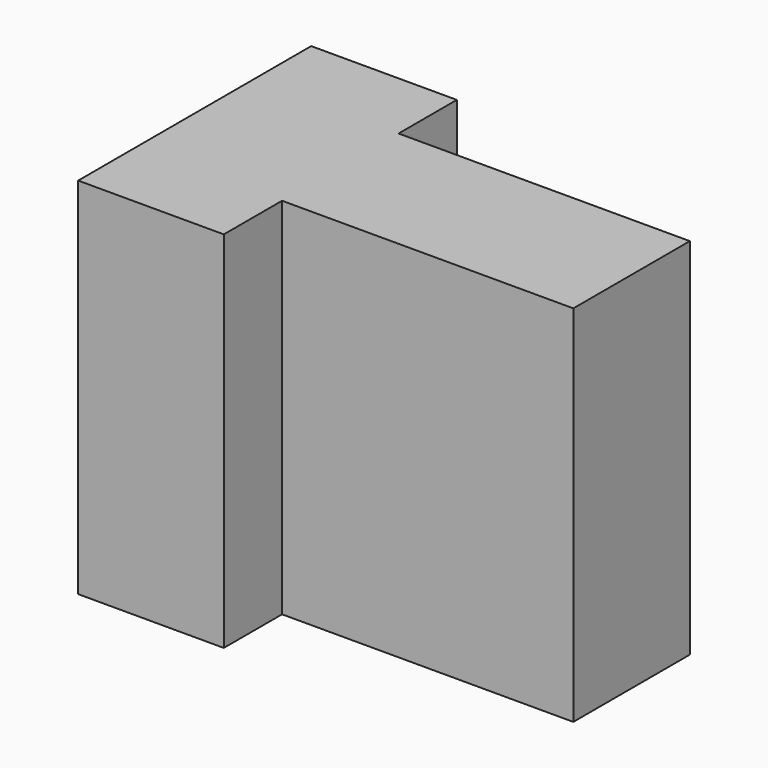
from build123d import *

# Parameters (mm, degrees)
F0_W     = 38.1
F0_H     = 31.75
F1_DEPTH = 25.4
F2_W     = 25.4
F2_H     = 31.75
F3_DEPTH = 6.35
F4_W     = 25.4
F4_H     = 31.75
F5_DEPTH = 6.35


# Not quite as in the source:
# - a feature names something its author has since deleted; it is built from what else it names


with BuildPart() as f1:
    # F0 (on Front) → F1 (new body)
    with BuildSketch(Plane.XZ):
        with Locations((-37.3860847076, 16.0793865216)):
            Rectangle(F0_W, F0_H)
    extrude(amount=F1_DEPTH)

    # F2 (on face) → F3 (cut)
    with BuildSketch(Plane.XZ.offset(25.4)):
        with Locations((-31.0360847076, 16.0793865216)):
            Rectangle(F2_W, F2_H)
    extrude(amount=-F3_DEPTH, mode=Mode.SUBTRACT)

    # F4 (on face) → F5 (cut)
    with BuildSketch(Plane(origin=(0, 0, 0), x_dir=(-1, 0, 0), z_dir=(0, 1, 0))):
        with Locations((31.0360847076, 16.0793865216)):
            Rectangle(F4_W, F4_H)
    extrude(amount=-F5_DEPTH, mode=Mode.SUBTRACT)


solid = f1.part
